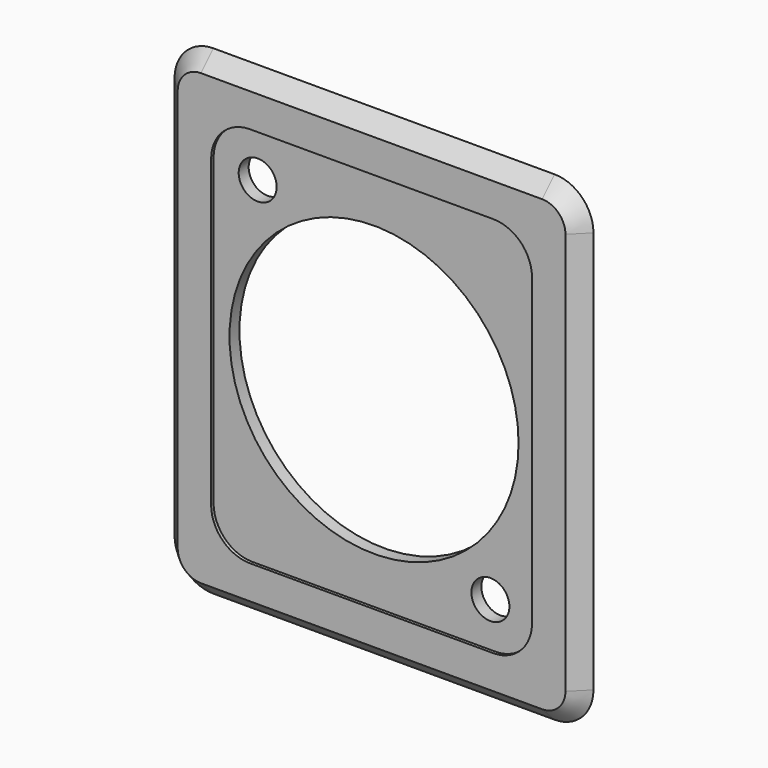
from build123d import *

# Parameters (mm, degrees)
F0_R     = 1.55
F0_R_2   = 11.8
F1_DEPTH = 1.27
F3_DEPTH = 0.254
F4_SIZE  = 1.26999


# Not quite as in the source:
# - a fillet or chamfer is up to 0.001 mm smaller than in the source, because OpenCascade refuses the exact size


with BuildPart() as f1:
    # F0 (on Front) → F1 (new body)
    with BuildSketch(Plane.XZ):
        with BuildLine():
            ThreePointArc((0, 3.175), (0.9299359697, 0.9299359697), (3.175, 0))
            Line((3.175, 0), (31.025, 0))
            ThreePointArc((31.025, 0), (33.2700640303, 0.9299359697), (34.2, 3.175))
            Line((34.2, 3.175), (34.2, 36.025))
            ThreePointArc((34.2, 36.025), (33.2700640303, 38.2700640303), (31.025, 39.2))
            Line((31.025, 39.2), (3.175, 39.2))
            ThreePointArc((3.175, 39.2), (0.9299359697, 38.2700640303), (0, 36.025))
            Line((0, 36.025), (0, 3.175))
        make_face()
        with Locations((26.5996, 7.6112)):
            Circle(F0_R, mode=Mode.SUBTRACT)
        with Locations((7.6004, 31.5888)):
            Circle(F0_R, mode=Mode.SUBTRACT)
        with Locations((17.1, 19.6)):
            Circle(F0_R_2, mode=Mode.SUBTRACT)
    extrude(amount=F1_DEPTH)

    # F2 (on face) → F3 (cut)
    with BuildSketch(Plane.XZ.offset(1.27)):
        with BuildLine():
            Line((27.025, 35.2), (7.175, 35.2))
            ThreePointArc((7.175, 35.2), (4.9299359697, 34.2700640303), (4, 32.025))
            Line((4, 32.025), (4, 7.175))
            ThreePointArc((4, 7.175), (4.9299359697, 4.9299359697), (7.175, 4))
            Line((7.175, 4), (27.025, 4))
            ThreePointArc((27.025, 4), (29.2700640303, 4.9299359697), (30.2, 7.175))
            Line((30.2, 7.175), (30.2, 32.025))
            ThreePointArc((30.2, 32.025), (29.2700640303, 34.2700640303), (27.025, 35.2))
        make_face()
    extrude(amount=-F3_DEPTH, mode=Mode.SUBTRACT)

    # F4 (size 1.27 in the source; OpenCascade refuses exactly that, so slightly less here)
    f4_edges = [f1.edges().sort_by_distance(p)[0] for p in [
        (34.2, -1.27, 19.6),
    ]]
    chamfer(f4_edges, length=F4_SIZE)


solid = f1.part
